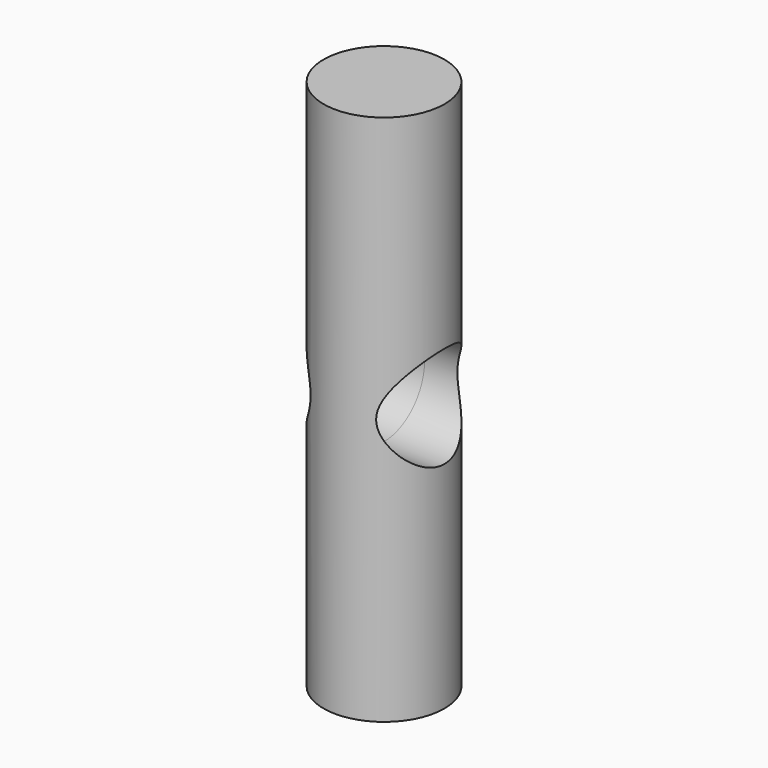
from build123d import *

# Parameters (mm, degrees)
F0_R          = 25
F1_DEPTH      = 110
F1_DEPTH_BACK = 110
F2_R          = 21
F3_DEPTH      = 25
F3_DEPTH_BACK = 25


# Not quite as in the source:
# - the program builds the solid bodies; features that only make, move or delete a surface that nothing else refers to are left out


with BuildPart() as f1:
    # F0 (on Top) → F1 (new body, two sides)
    with BuildSketch(Plane.XY) as f1_sk:
        Circle(F0_R)
    extrude(amount=F1_DEPTH)
    extrude(f1_sk.sketch, amount=-F1_DEPTH_BACK)

    # F2 (on Right) → F3 (cut, two sides)
    with BuildSketch(Plane.YZ) as f3_sk:
        Circle(F2_R)
    extrude(amount=F3_DEPTH, mode=Mode.SUBTRACT)
    extrude(f3_sk.sketch, amount=-F3_DEPTH_BACK, mode=Mode.SUBTRACT)


solid = f1.part
